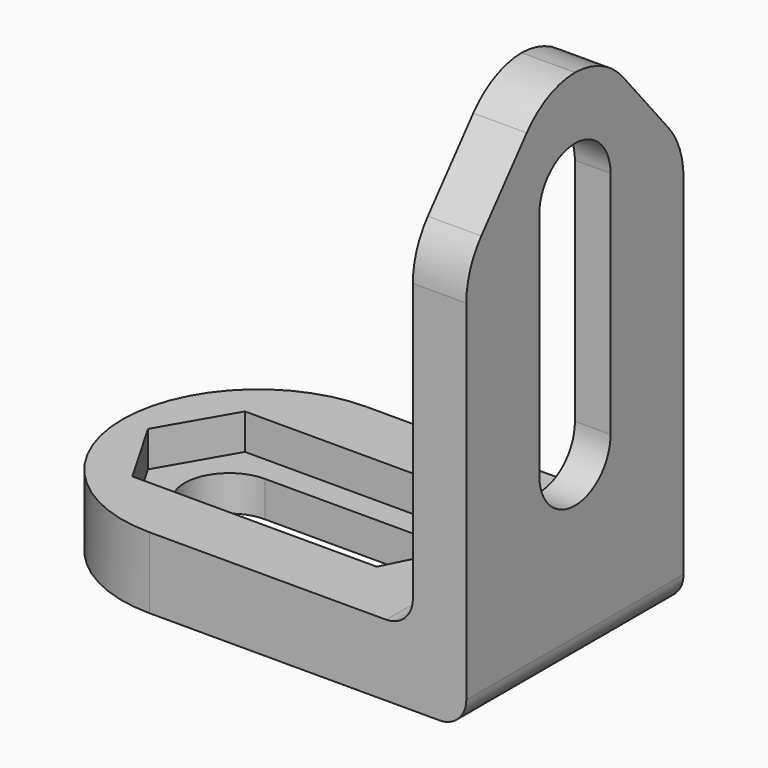
from build123d import *

# Parameters (mm, degrees)
F1_DEPTH    = 15.24
F3_DEPTH    = 1
F4_DEPTH    = 3
F6_DEPTH    = 2
F7_DEPTH    = 4
F8_SIZE2    = 6.6595190754
F8_SIZE     = 5.588
F9_T1_DEPTH = 11.189330271
F9_T3_DEPTH = 13.4919223085
F10_R       = 7.61999


# Not quite as in the source:
# - a fillet or chamfer that OpenCascade refuses, or shapes differently, is made with other operations: its cross-section is extruded or revolved along the edge and cut away or added
# - a fillet or chamfer is up to 0.001 mm smaller than in the source, because OpenCascade refuses the exact size


with BuildPart() as f1:
    # F0 (on Front) → F1 (new body)
    with BuildSketch(Plane.XZ):
        with BuildLine():
            ThreePointArc((-3, 4.5), (-3.4393398282, 3.4393398282), (-4.5, 3))
            Line((-4.5, 3), (-25.4, 3))
            Line((-25.4, 3), (-25.4, -1))
            Line((-25.4, -1), (-1.5, -1))
            ThreePointArc((-1.5, -1), (-0.4393398282, -0.5606601718), (0, 0.5))
            Line((0, 0.5), (0, 28.4))
            Line((0, 28.4), (-3, 28.4))
            Line((-3, 28.4), (-3, 4.5))
        make_face()
    extrude(amount=F1_DEPTH)

    # F2 (on face) → F3 (cut)
    with BuildSketch(Plane(origin=(-3, 0, 0), x_dir=(0, -1, 0), z_dir=(-1, 0, 0))):
        Polygon((11.57, 20.1194664367), (11.57, 22.4), (11.57, 24.6805335633), (7.62, 26.9610671266), (3.67, 24.6805335633), (3.67, 22.4), (3.67, 20.1194664367), (3.67, 11.7805335633), (3.67, 9.5), (3.67, 7.2194664367), (7.62, 4.9389328734), (11.57, 7.2194664367), (11.57, 9.5), (11.57, 11.7805335633), align=None)
        with BuildLine():
            Line((5.12, 9.5), (5.12, 22.4))
            ThreePointArc((5.12, 22.4), (7.62, 24.9), (10.12, 22.4))
            Line((10.12, 22.4), (10.12, 9.5))
            ThreePointArc((10.12, 9.5), (7.62, 7), (5.12, 9.5))
        make_face(mode=Mode.SUBTRACT)
    extrude(amount=-F3_DEPTH, mode=Mode.SUBTRACT)

    # F4 (cut, through all): a face of the model
    f4_faces = [f1.faces().sort_by_distance(p)[0] for p in [
        (-3, -7.62, 15.95),
    ]]
    extrude(f4_faces, amount=-F4_DEPTH, mode=Mode.SUBTRACT)

    # F5 (on face) → F6 (cut)
    with BuildSketch(Plane.XY.offset(3)):
        Polygon((-21.6805335633, -11.57), (-7.9645335633, -11.57), (-5.938922, -7.52), (-7.9645335633, -3.67), (-21.6805335633, -3.67), (-23.9610671266, -7.62), align=None)
        with BuildLine():
            Line((-10.5, -10.12), (-19.4, -10.12))
            ThreePointArc((-19.4, -10.12), (-21.9, -7.62), (-19.4, -5.12))
            Line((-19.4, -5.12), (-10.5, -5.12))
            ThreePointArc((-10.5, -5.12), (-8, -7.62), (-10.5, -10.12))
        make_face(mode=Mode.SUBTRACT)
    extrude(amount=-F6_DEPTH, mode=Mode.SUBTRACT)

    # F7 (cut, through all): a face of the model
    f7_faces = [f1.faces().sort_by_distance(p)[0] for p in [
        (-14.95, -7.62, 3),
    ]]
    extrude(f7_faces, amount=-F7_DEPTH, mode=Mode.SUBTRACT)

    # F8
    f8_edges = [f1.edges().sort_by_distance(p)[0] for p in [
        (-1.5, -15.24, 28.4),
        (-1.5, 0, 28.4),
    ]]
    f8_side = f1.faces().sort_by_distance((-1.5, -7.62, 28.4))[0]
    chamfer(f8_edges, length=F8_SIZE, length2=F8_SIZE2, reference=f8_side)

    # F9: fillet of radius 4.5 on 4 edges, made by hand

    # F9_s2 → F9_t1 (cut)
    with BuildSketch(Plane.YZ.offset(-7.0946651355)):
        with BuildLine():
            ThreePointArc((-14.187199994, 22.995159114), (-14.9686167935, 21.6417055154), (-15.24, 20.1026148704))
            Line((-15.24, 20.1026148704), (-15.24, 21.7404809246))
            Line((-15.24, 21.7404809246), (-14.187199994, 22.995159114))
        make_face()
        with BuildLine():
            ThreePointArc((-1.052800006, 22.995159114), (-0.2713832065, 21.6417055154), (0, 20.1026148704))
            Line((0, 20.1026148704), (0, 21.7404809246))
            Line((0, 21.7404809246), (-1.052800006, 22.995159114))
        make_face()
    extrude(amount=F9_T1_DEPTH, mode=Mode.SUBTRACT)

    # F9_s4 → F9_t3 (cut)
    with BuildSketch(Plane.YZ.offset(-8.2459611542)):
        with BuildLine():
            ThreePointArc((-7.5536155383, 28.4), (-9.4553977161, 27.9783850417), (-11.0008155323, 26.7925442436))
            Line((-11.0008155323, 26.7925442436), (-9.652, 28.4))
            Line((-9.652, 28.4), (-7.5536155383, 28.4))
        make_face()
        with BuildLine():
            ThreePointArc((-7.6863844617, 28.4), (-5.7846022839, 27.9783850417), (-4.2391844677, 26.7925442436))
            Line((-4.2391844677, 26.7925442436), (-5.588, 28.4))
            Line((-5.588, 28.4), (-7.6863844617, 28.4))
        make_face()
    extrude(amount=F9_T3_DEPTH, mode=Mode.SUBTRACT)

    # F10 (radius 7.62 in the source; OpenCascade refuses exactly that, so slightly less here)
    f10_edges = [f1.edges().sort_by_distance(p)[0] for p in [
        (-25.4, -15.24, 1),
        (-25.4, 0, 1),
    ]]
    fillet(f10_edges, radius=F10_R)


solid = f1.part
